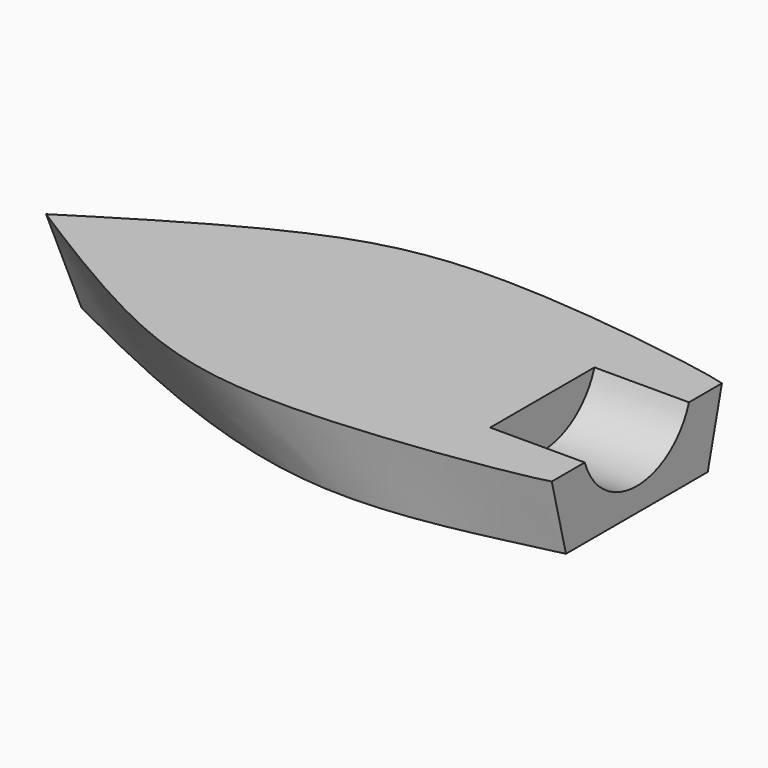
from build123d import *

# Parameters (mm, degrees)
F5_DEPTH = 40


with BuildPart() as f3:
    # F2 (on offset) → F3 section 0
    with BuildSketch(Plane.XY.offset(-30)):
        with BuildLine():
            Line((162.2463304921, -37.5), (162.2463304921, 0))
            Line((162.2463304921, 0), (162.2463304921, 37.5))
            add(Edge.make_bspline(
                [(-72.7536695079, 0), (-29.5158392356, 21.6682380863), (60.1620321507, 64.9393967263), (129.9707958681, 44.834202262), (162.2463304921, 37.5)],
                knots=[0, 0, 0, 0, 0.5444604727, 1, 1, 1, 1], degree=3))
            add(Edge.make_bspline(
                [(-72.7536695079, 0), (-29.5158392356, -21.6682380863), (60.1620321507, -64.9393967263), (129.9707958681, -44.834202262), (162.2463304921, -37.5)],
                knots=[0, 0, 0, 0, 0.5444604727, 1, 1, 1, 1], degree=3))
        make_face()
    # F0 (on Top) → F3 section 1
    with BuildSketch(Plane.XY):
        with BuildLine():
            Line((162.2463304921, -45), (162.2463304921, 0))
            Line((162.2463304921, 0), (162.2463304921, 45))
            add(Edge.make_bspline(
                [(162.2463304921, 45), (150.1698760976, 48.6930710105), (52.7402528222, 64.2426959064), (-14.1104264901, 47.0441984602), (-73.803611279, 8.7933518628), (-87.7536695079, 0)],
                knots=[0, 0, 0, 0, 0.3575982232, 0.6819644283, 1, 1, 1, 1], degree=3))
            add(Edge.make_bspline(
                [(162.2463304921, -45), (150.1698760976, -48.6930710105), (52.7402528222, -64.2426959064), (-14.1104264901, -47.0441984602), (-73.803611279, -8.7933518628), (-87.7536695079, 0)],
                knots=[0, 0, 0, 0, 0.3575982232, 0.6819644283, 1, 1, 1, 1], degree=3))
        make_face()
    loft()

    # F4 (on face) → F5 (cut)
    with BuildSketch(Plane.YZ.offset(162.2463304921)):
        with BuildLine():
            Line((27.5680975042, 0), (-27.5680975042, 0))
            ThreePointArc((-27.5680975042, 0), (0, -20), (27.5680975042, 0))
        make_face()
    extrude(amount=-F5_DEPTH, mode=Mode.SUBTRACT)


solid = f3.part
